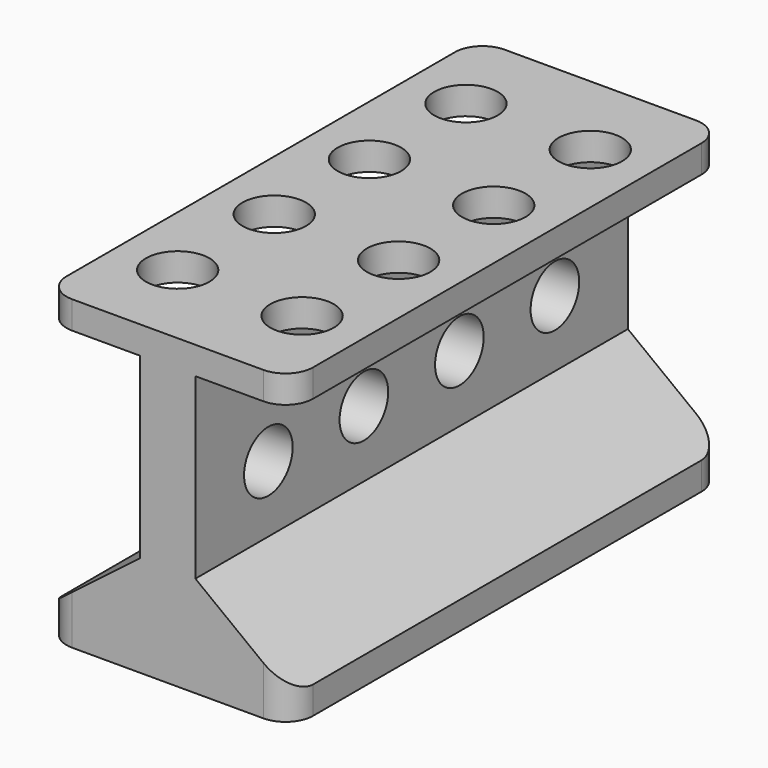
from build123d import *

# Parameters (mm, degrees)
F1_DEPTH = 48.9
F3_R     = 5
F5_D     = 11
F7_D     = 11.5
F7_DEPTH = 12
F7_TIP   = 3.4549485594


# Not quite as in the source:
# - a feature names something its author has since deleted; it is built from what else it names


with BuildPart() as f1:
    # F0 (on Front) → F1 (new body, symmetric)
    with BuildSketch(Plane.XZ):
        Polygon((-5, 20.25), (5, 20.25), (22.3, 20.25), (22.3, 25.25), (-22.3, 25.25), (-22.3, 20.25), align=None)
        Polygon((5, 0), (5, 20.25), (-5, 20.25), (-5, -12), (-5, -20.25), (0, -20.25), (5, -20.25), (5, -12), align=None)
        Polygon((-5, -20.25), (-5, -12), (-22.3, -25.25), (-22.3, -30.25), (22.3, -30.25), (22.3, -25.25), (5, -12), (5, -20.25), (0, -20.25), align=None)
    extrude(amount=F1_DEPTH, both=True)

    # F3
    f3_edges = [f1.edges().sort_by_distance(p)[0] for p in [
        (-22.3, 48.9, 22.75),
        (-22.3, -48.9, 22.75),
        (22.3, 48.9, 22.75),
        (22.3, -48.9, 22.75),
        (-22.3, -48.9, -27.75),
        (22.3, -48.9, -27.75),
        (-22.3, 48.9, -27.75),
        (22.3, 48.9, -27.75),
    ]]
    fillet(f3_edges, radius=F3_R)

    # F5 (through all)
    with Locations(Plane(origin=(-5, 0, 0), x_dir=(0, -1, 0), z_dir=(-1, 0, 0))):
        with Locations((32.4, 0), (10.8, 0), (-10.8, 0), (-32.4, 0)):
            Hole(F5_D / 2)

    # F7
    with Locations(Plane.XY.offset(25.25)):
        with Locations((-11.25, 32.5910784304), (11.25, 32.5910784304), (11.25, 10.7566630468), (-11.25, 10.7566630468), (-11.25, -10.7566630468), (11.25, -10.7566630468), (11.25, -32.5910784304), (-11.25, -32.5910784304)):
            Hole(F7_D / 2, depth=F7_DEPTH)
            with Locations((0, 0, -(F7_DEPTH + F7_TIP / 2))):  # 118° drill point
                Cone(0, F7_D / 2, F7_TIP, mode=Mode.SUBTRACT)


solid = f1.part
